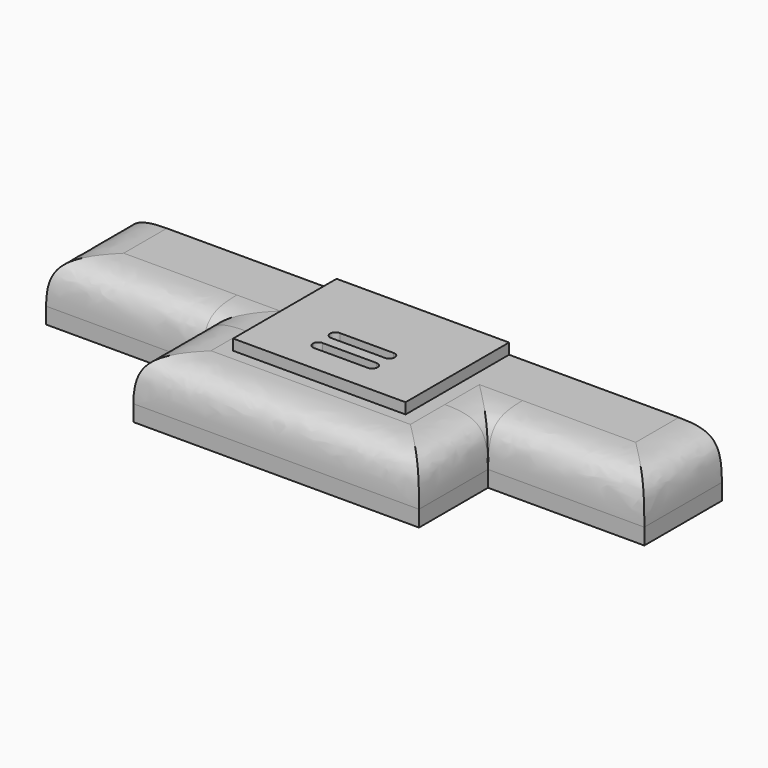
from build123d import *

# Parameters (mm, degrees)
F1_DEPTH     = 5.5
F2_T1_DEPTH  = 24.5
F2_T3_DEPTH  = 29
F2_T5_DEPTH  = 46.5
F2_T7_DEPTH  = 18
F2_T9_DEPTH  = 24.5
F2_T15_DEPTH = 34.5
F2_T19_DEPTH = 28
F2_T26_DEPTH = 28
F2_T30_DEPTH = 34.5
F3_W         = 16
F3_H         = 12
F4_DEPTH     = 1
F6_DEPTH     = 1.5


# Not quite as in the source:
# - a fillet or chamfer that OpenCascade refuses, or shapes differently, is made with other operations: its cross-section is extruded or revolved along the edge and cut away or added


with BuildPart() as f1:
    # F0 (on Top) → F1 (new body)
    with BuildSketch(Plane.XY):
        Polygon((55.5, 0), (0, 0), (0, -9), (14.5, -9), (14.5, -17), (41, -17), (41, -9), (55.5, -9), align=None)
    extrude(amount=F1_DEPTH)

    # F2: fillet of radius 4 on 7 edges, made by hand

    # F2_s2 → F2_t1 (cut)
    with BuildSketch(Plane.YZ.offset(-10)):
        with BuildLine():
            add(Edge.make_bspline(
                [(-9, 1.5), (-9, 5.5), (-5, 5.5)],
                knots=[0, 0, 0, 1, 1, 1], degree=2, weights=[1, 1.5, 1]))
            Line((-5, 5.5), (-9, 5.5))
            Line((-9, 5.5), (-9, 1.5))
        make_face()
    extrude(amount=F2_T1_DEPTH, mode=Mode.SUBTRACT)

    # F2_s4 → F2_t3 (cut)
    with BuildSketch(Plane.XZ.offset(-10)):
        with BuildLine():
            add(Edge.make_bspline(
                [(0, 1.5), (0, 5.5), (4, 5.5)],
                knots=[0, 0, 0, 1, 1, 1], degree=2, weights=[1, 1.5, 1]))
            Line((4, 5.5), (0, 5.5))
            Line((0, 5.5), (0, 1.5))
        make_face()
        with BuildLine():
            add(Edge.make_bspline(
                [(55.5, 1.5), (55.5, 5.5), (51.5, 5.5)],
                knots=[0, 0, 0, 1, 1, 1], degree=2, weights=[1, 1.5, 1]))
            Line((51.5, 5.5), (55.5, 5.5))
            Line((55.5, 5.5), (55.5, 1.5))
        make_face()
    extrude(amount=F2_T3_DEPTH, mode=Mode.SUBTRACT)

    # F2_s6 → F2_t5 (cut)
    with BuildSketch(Plane.YZ.offset(4.5)):
        with BuildLine():
            add(Edge.make_bspline(
                [(-17, 1.5), (-17, 5.5), (-13, 5.5)],
                knots=[0, 0, 0, 1, 1, 1], degree=2, weights=[1, 1.5, 1]))
            Line((-13, 5.5), (-17, 5.5))
            Line((-17, 5.5), (-17, 1.5))
        make_face()
    extrude(amount=F2_T5_DEPTH, mode=Mode.SUBTRACT)

    # F2_s8 → F2_t7 (cut)
    with BuildSketch(Plane.XZ.offset(9)):
        with BuildLine():
            add(Edge.make_bspline(
                [(41, 1.5), (41, 5.5), (37, 5.5)],
                knots=[0, 0, 0, 1, 1, 1], degree=2, weights=[1, 1.5, 1]))
            Line((37, 5.5), (41, 5.5))
            Line((41, 5.5), (41, 1.5))
        make_face()
        with BuildLine():
            add(Edge.make_bspline(
                [(14.5, 1.5), (14.5, 5.5), (18.5, 5.5)],
                knots=[0, 0, 0, 1, 1, 1], degree=2, weights=[1, 1.5, 1]))
            Line((18.5, 5.5), (14.5, 5.5))
            Line((14.5, 5.5), (14.5, 1.5))
        make_face()
    extrude(amount=F2_T7_DEPTH, mode=Mode.SUBTRACT)

    # F2_s10 → F2_t9 (cut)
    with BuildSketch(Plane.YZ.offset(41)):
        with BuildLine():
            add(Edge.make_bspline(
                [(-9, 1.5), (-9, 5.5), (-5, 5.5)],
                knots=[0, 0, 0, 1, 1, 1], degree=2, weights=[1, 1.5, 1]))
            Line((-5, 5.5), (-9, 5.5))
            Line((-9, 5.5), (-9, 1.5))
        make_face()
    extrude(amount=F2_T9_DEPTH, mode=Mode.SUBTRACT)


with BuildPart() as f2_tool13:
    # F2_s14 → F2_t15 (new body)
    with BuildSketch(Plane.YZ.offset(-10)):
        with BuildLine():
            add(Edge.make_bspline(
                [(-9, 1.5), (-9, 5.5), (-5, 5.5)],
                knots=[0, 0, 0, 1, 1, 1], degree=2, weights=[1, 1.5, 1]))
            Line((-5, 5.5), (-9, 5.5))
            Line((-9, 5.5), (-9, 1.5))
        make_face()
    extrude(amount=F2_T15_DEPTH)

    split(bisect_by=Plane.YZ.offset(14.5), keep=Keep.TOP)


with BuildPart() as f2_tool17:
    # F2_s18 → F2_t19 (new body)
    with BuildSketch(Plane.XZ.offset(-1)):
        with BuildLine():
            add(Edge.make_bspline(
                [(14.5, 1.5), (14.5, 5.5), (18.5, 5.5)],
                knots=[0, 0, 0, 1, 1, 1], degree=2, weights=[1, 1.5, 1]))
            Line((18.5, 5.5), (14.5, 5.5))
            Line((14.5, 5.5), (14.5, 1.5))
        make_face()
    extrude(amount=F2_T19_DEPTH)

    split(bisect_by=Plane.XZ.offset(9), keep=Keep.BOTTOM)


with BuildPart() as f2_tool13_1:
    add(f2_tool13.part)

    # F2_t21: intersect F2_tool17
    add(f2_tool17.part, mode=Mode.INTERSECT)


with BuildPart() as f1_1:
    add(f1.part)

    # F2_t11: cut F2_tool13
    add(f2_tool13_1.part, mode=Mode.SUBTRACT)


with BuildPart() as f2_tool24:
    # F2_s25 → F2_t26 (new body)
    with BuildSketch(Plane.XZ.offset(27)):
        with BuildLine():
            add(Edge.make_bspline(
                [(41, 1.5), (41, 5.5), (37, 5.5)],
                knots=[0, 0, 0, 1, 1, 1], degree=2, weights=[1, 1.5, 1]))
            Line((37, 5.5), (41, 5.5))
            Line((41, 5.5), (41, 1.5))
        make_face()
    extrude(amount=-F2_T26_DEPTH)

    split(bisect_by=Plane.XZ.offset(9), keep=Keep.BOTTOM)


with BuildPart() as f2_tool28:
    # F2_s29 → F2_t30 (new body)
    with BuildSketch(Plane.YZ.offset(31)):
        with BuildLine():
            add(Edge.make_bspline(
                [(-9, 1.5), (-9, 5.5), (-5, 5.5)],
                knots=[0, 0, 0, 1, 1, 1], degree=2, weights=[1, 1.5, 1]))
            Line((-5, 5.5), (-9, 5.5))
            Line((-9, 5.5), (-9, 1.5))
        make_face()
    extrude(amount=F2_T30_DEPTH)

    split(bisect_by=Plane.YZ.offset(41), keep=Keep.BOTTOM)


with BuildPart() as f2_tool24_1:
    add(f2_tool24.part)

    # F2_t32: intersect F2_tool28
    add(f2_tool28.part, mode=Mode.INTERSECT)


with BuildPart() as f1_2:
    add(f1_1.part)

    # F2_t22: cut F2_tool24
    add(f2_tool24_1.part, mode=Mode.SUBTRACT)

    # F3 (on face) → F4 (join)
    with BuildSketch(Plane.XY.offset(5.5)):
        with Locations((27.75, -6)):
            Rectangle(F3_W, F3_H)
    extrude(amount=F4_DEPTH)

    # F5 (on face) → F6 (cut)
    with BuildSketch(Plane.XY.offset(6.5)):
        with BuildLine():
            ThreePointArc((25.25, -6.5), (24.75, -7), (25.25, -7.5))
            Line((25.25, -7.5), (30.25, -7.5))
            ThreePointArc((30.25, -7.5), (30.75, -7), (30.25, -6.5))
            Line((30.25, -6.5), (25.25, -6.5))
        make_face()
        with BuildLine():
            Line((30.25, -9), (25.25, -9))
            Line((25.25, -9), (24.75, -9))
            ThreePointArc((24.75, -9), (24.8964466094, -9.3535533906), (25.25, -9.5))
            Line((25.25, -9.5), (30.25, -9.5))
            ThreePointArc((30.25, -9.5), (30.6035533906, -9.3535533906), (30.75, -9))
            Line((30.75, -9), (30.25, -9))
        make_face()
        with BuildLine():
            Line((24.75, -9), (25.25, -9))
            Line((25.25, -9), (30.25, -9))
            Line((30.25, -9), (30.75, -9))
            ThreePointArc((30.75, -9), (30.6035533906, -8.6464466094), (30.25, -8.5))
            Line((30.25, -8.5), (25.25, -8.5))
            ThreePointArc((25.25, -8.5), (24.8964466094, -8.6464466094), (24.75, -9))
        make_face()
    extrude(amount=-F6_DEPTH, mode=Mode.SUBTRACT)


solid = f1_2.part
